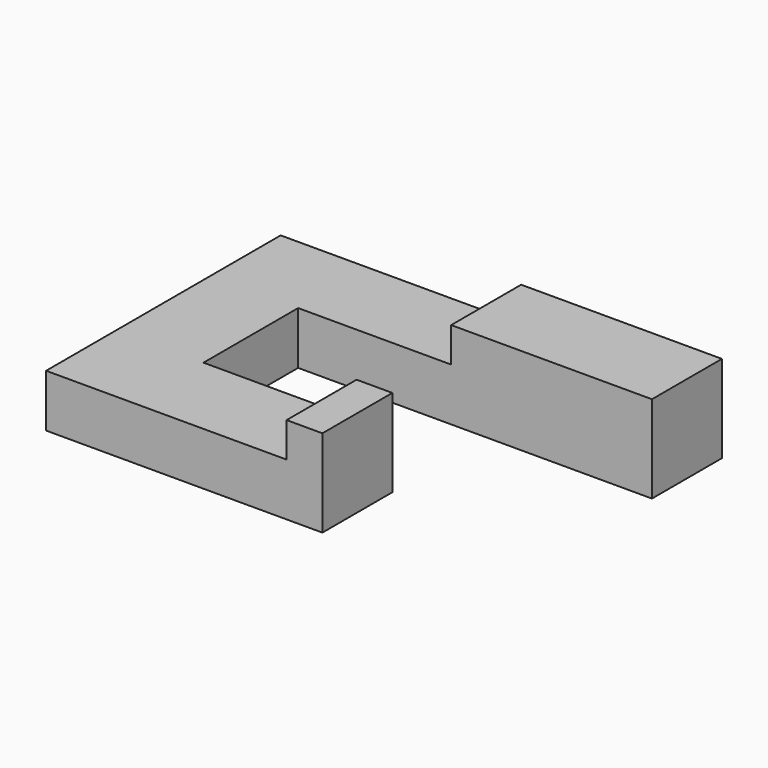
from build123d import *

# Parameters (mm, degrees)
F0_W     = 977.9
F0_H     = 558.8
F4_DEPTH = 336.55
F0_W_2   = 228.6
F0_W_3   = 1282.7
F5_DEPTH = 558.8


# Not quite as in the source:
# - the program builds the solid bodies; features that only make, move or delete a surface that nothing else refers to are left out


with BuildPart() as f4:
    # F0 (on Top) → F4 (new body)
    with BuildSketch(Plane.XY):
        with Locations((-361.95, -657.225)):
            Rectangle(F0_W, F0_H)
        with Locations((-361.95, 657.225)):
            Rectangle(F0_W, F0_H)
        Polygon((-850.9, 936.625), (-1409.7, 936.625), (-1409.7, -936.625), (-850.9, -936.625), (-850.9, -377.825), (-850.9, 377.825), align=None)
    extrude(amount=F4_DEPTH)

    # F0 (on Top) → F5 (join)
    with BuildSketch(Plane.XY):
        with Locations((241.3, -657.225)):
            Rectangle(F0_W_2, F0_H)
        with Locations((768.35, 657.225)):
            Rectangle(F0_W_3, F0_H)
    extrude(amount=F5_DEPTH)


solid = f4.part
